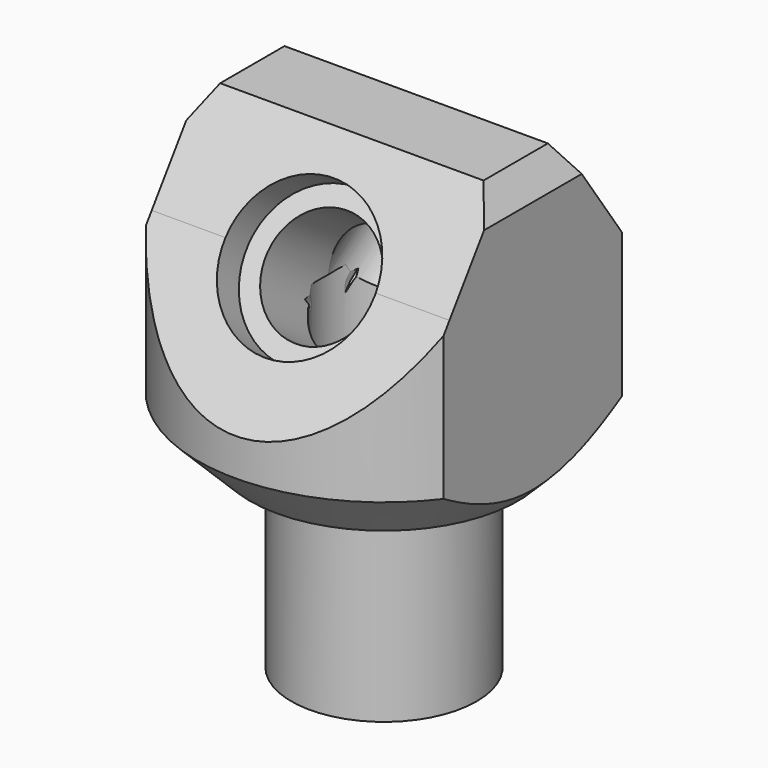
from build123d import *

# Parameters (mm, degrees)
F0_R        = 25
F1_DEPTH    = 65.5
F2_R        = 8
F3_DEPTH    = 44
F4_W        = 17.7049817399
F4_H        = 63.7933180105
F4_W_2      = 20.9798936745
F4_H_2      = 49.4306737048
F5_DEPTH    = 49.3
F6_C1_SIZE2 = 2.3094010768
F6_C1_SIZE  = 4
F6_C2_SIZE2 = 4
F6_C2_SIZE  = 2.3094010768
F7_R        = 27.6347360806
F7_R_2      = 12.45
F8_DEPTH    = 25.5
F9_R        = 2
F11_DEPTH   = 44.3
F12_C1_SIZE = 7
F12_C2_SIZE = 6.9999
F13_R       = 10.1
F14_DEPTH   = 4.5
F15_R       = 10.1
F16_DEPTH   = 4.5
F17_R       = 7.5
F18_DEPTH   = 16.5
F19_R       = 7.5
F20_DEPTH   = 16.5


# Not quite as in the source:
# - a fillet or chamfer is up to 0.001 mm smaller than in the source, because OpenCascade refuses the exact size


with BuildPart() as f1:
    # F0 (on Top) → F1 (new body)
    with BuildSketch(Plane.XY):
        Circle(F0_R)
    extrude(amount=F1_DEPTH)

    # F2 (on face) → F3 (cut)
    with BuildSketch(Plane(origin=(0, 0, 0), x_dir=(1, 0, 0), z_dir=(0, 0, -1))):
        Circle(F2_R)
    extrude(amount=-F3_DEPTH, mode=Mode.SUBTRACT)

    # F4 (on Front) → F5 (cut, symmetric)
    with BuildSketch(Plane.XZ):
        with Locations((28.8524908699, 55.8966590053)):
            Rectangle(F4_W, F4_H)
        with Locations((-30.4899468372, 48.7153368524)):
            Rectangle(F4_W_2, F4_H_2)
    extrude(amount=F5_DEPTH, both=True, mode=Mode.SUBTRACT)

    # F6: chamfer of 4 x 2.3094010768 on 2 edges, made by hand

    # F6_c1
    f6_c1_edges = [f1.edges().sort_by_distance(p)[0] for p in [
        (20, 0, 65.5),
    ]]
    f6_c1_side = f1.faces().sort_by_distance((20, 0, 65.4538119785))[0]
    chamfer(f6_c1_edges, length=F6_C1_SIZE, length2=F6_C1_SIZE2, reference=f6_c1_side)

    # F6_c2
    f6_c2_edges = [f1.edges().sort_by_distance(p)[0] for p in [
        (-20, 0, 65.5),
    ]]
    f6_c2_side = f1.faces().sort_by_distance((-19.9538119785, 0, 65.5))[0]
    chamfer(f6_c2_edges, length=F6_C2_SIZE, length2=F6_C2_SIZE2, reference=f6_c2_side)

    # F7 (on face) → F8 (cut)
    with BuildSketch(Plane(origin=(0, 0, 0), x_dir=(1, 0, 0), z_dir=(0, 0, -1))):
        Circle(F7_R)
        Circle(F7_R_2, mode=Mode.SUBTRACT)
    extrude(amount=-F8_DEPTH, mode=Mode.SUBTRACT)

    # F9
    f9_edges = [f1.edges().sort_by_distance(p)[0] for p in [
        (-12.45, 0, 25.5),
    ]]
    fillet(f9_edges, radius=F9_R)

    # F10 (on Right) → F11 (cut, symmetric)
    with BuildSketch(Plane.YZ):
        Polygon((2.7942564781, 69.2223283856), (14.0074999573, 53.2081570616), (27.8284827581, 33.4697480234), (27.8284827581, 71.2105557323), align=None)
        Polygon((-28.691531344, 32.2371869058), (-14.0074999573, 53.2081570616), (-2.0273737507, 70.3175504242), (-27.1908640862, 71.7121362686), align=None)
    extrude(amount=F11_DEPTH, both=True, mode=Mode.SUBTRACT)

    # F12: chamfer of 7 on 3 edges, made by hand

    # F12_c1
    f12_c1_edges = [f1.edges().sort_by_distance(p)[0] for p in [
        (0, 25, 25.5),
    ]]
    chamfer(f12_c1_edges, length=F12_C1_SIZE)

    # F12_c2 (size 7 in the source; OpenCascade refuses exactly that, so slightly less here)
    f12_c2_edges = [f1.edges().sort_by_distance(p)[0] for p in [
        (0, -25, 25.5),
    ]]
    chamfer(f12_c2_edges, length=F12_C2_SIZE)

    # F13 (on face) → F14 (cut)
    with BuildSketch(Plane(origin=(0, -34.3988298284, 24.0863199514), x_dir=(1, 0, 0), z_dir=(0, -0.8191520443, 0.5735764364))):
        with Locations((0, 35.2567682304)):
            Circle(F13_R)
    extrude(amount=-F14_DEPTH, mode=Mode.SUBTRACT)

    # F15 (on face) → F16 (cut)
    with BuildSketch(Plane(origin=(0, 34.3988298284, 24.0863199514), x_dir=(-1, 0, 0), z_dir=(0, 0.8191520443, 0.5735764364))):
        with Locations((0, 35.2567682304)):
            Circle(F15_R)
    extrude(amount=-F16_DEPTH, mode=Mode.SUBTRACT)

    # F17 (on face) → F18 (cut)
    with BuildSketch(Plane(origin=(0, 30.7126456291, 21.5052259879), x_dir=(-1, 0, 0), z_dir=(0, 0.8191520443, 0.5735764364))):
        with Locations((0, 35.2567682304)):
            Circle(F17_R)
    extrude(amount=-F18_DEPTH, mode=Mode.SUBTRACT)

    # F19 (on face) → F20 (cut)
    with BuildSketch(Plane(origin=(0, -30.7126456291, 21.5052259879), x_dir=(1, 0, 0), z_dir=(0, -0.8191520443, 0.5735764364))):
        with Locations((0, 35.2567682304)):
            Circle(F19_R)
    extrude(amount=-F20_DEPTH, mode=Mode.SUBTRACT)


solid = f1.part
